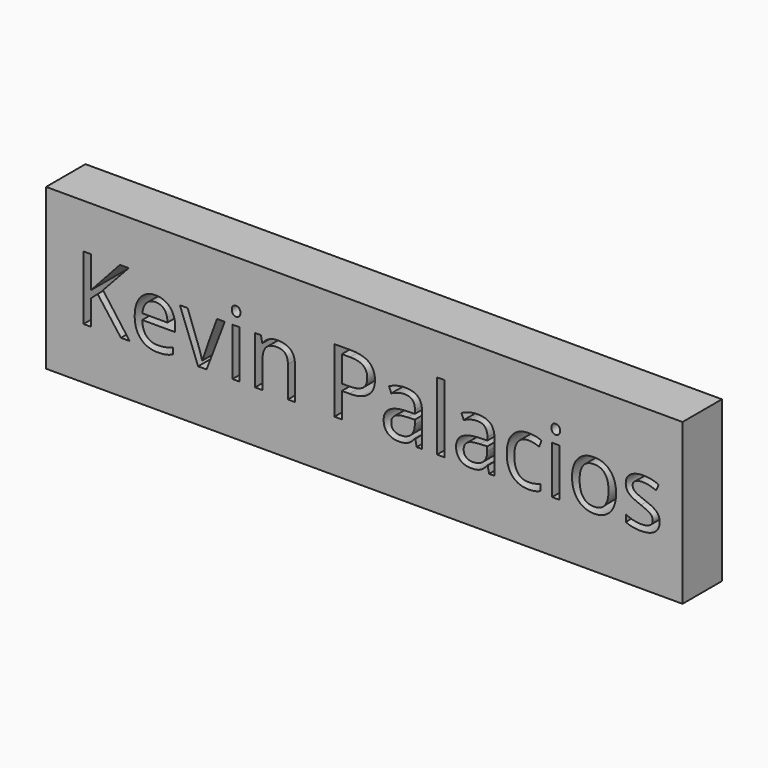
from build123d import *

# Parameters (mm, degrees)
F0_W         = 164.1767024994
F0_H         = 41.3037501276
F1_DEPTH     = 12.7
F2_TEXT_SIZE = 23.0958300774
F3_DEPTH     = 70.612


# Not quite as in the source:
# - Text() gives the source's letters only with a copy of the font that has no kerning and outlines rounded to 1/6400 em; it was checked with that copy


with BuildPart() as f1:
    # F0 (on Front) → F1 (new body)
    with BuildSketch(Plane.XZ):
        with Locations((15.6669840217, 48.9603746682)):
            Rectangle(F0_W, F0_H)
    extrude(amount=F1_DEPTH)

    # F2 (on Front) → F3 (cut)
    with BuildSketch(Plane.XZ):
        with Locations((-59.0343201022, 41.6103928816)):
            Text('Kevin Palacios', F2_TEXT_SIZE, font='Open Sans', text_align=(TextAlign.LEFT, TextAlign.BOTTOM))
    extrude(amount=F3_DEPTH, mode=Mode.SUBTRACT)


solid = f1.part
